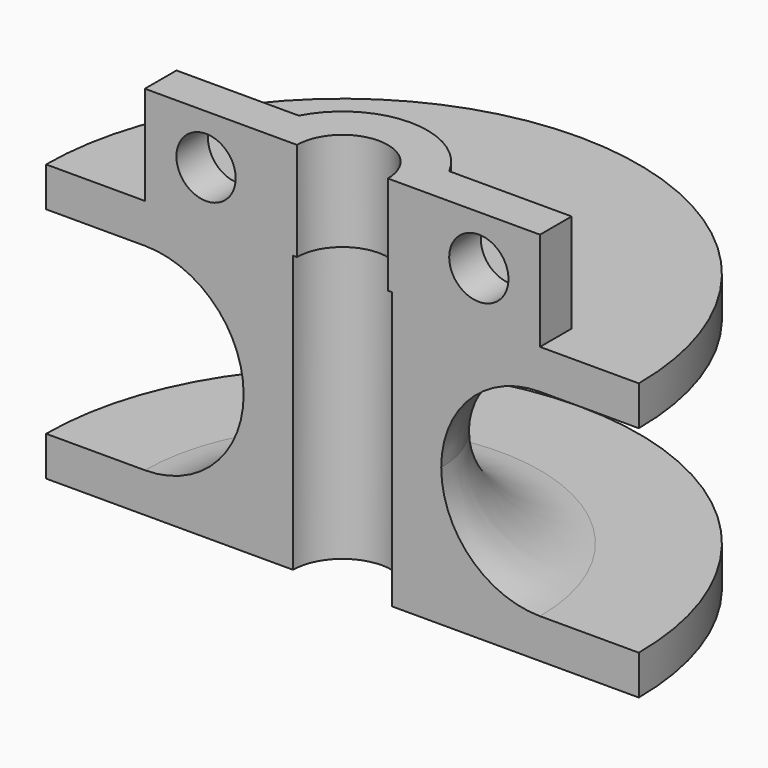
from build123d import *

# Parameters (mm, degrees)
F1_ANGLE = 180
F3_DEPTH = 5
F4_R     = 1.5
F5_DEPTH = 2.001
F6_R     = 4.99999


# Not quite as in the source:
# - a fillet or chamfer is up to 0.001 mm smaller than in the source, because OpenCascade refuses the exact size


with BuildPart() as f1:
    # F0 (on Front) → F1 (revolve)
    with BuildSketch(Plane.XZ):
        Polygon((-2.5, -7), (-2.5, 7), (-15, 7), (-15, 5), (-5, 5), (-5, -5), (-15, -5), (-15, -7), align=None)
    revolve(axis=Axis((0, 0, 0.6770828075), (0, 0, -1)), revolution_arc=F1_ANGLE)

    # F2 (on face) → F3 (join)
    with BuildSketch(Plane.XY.offset(7)):
        with BuildLine():
            Line((-10, 2), (-10, 0))
            Line((-10, 0), (-2.3, 0))
            ThreePointArc((-2.3, 0), (0, 2.3), (2.3, 0))
            Line((2.3, 0), (10, 0))
            Line((10, 0), (10, 2))
            Line((10, 2), (3.8065732621, 2))
            ThreePointArc((3.8065732621, 2), (0, 4.3), (-3.8065732621, 2))
            Line((-3.8065732621, 2), (-10, 2))
        make_face()
    extrude(amount=F3_DEPTH)

    # F4 (on face) → F5 (cut, through all)
    with BuildSketch(Plane(origin=(0, 2, 0), x_dir=(-1, 0, 0), z_dir=(0, 1, 0))):
        with Locations((6.9032866311, 9.5)):
            Circle(F4_R)
        with Locations((-6.9032866311, 9.5)):
            Circle(F4_R)
    extrude(amount=-F5_DEPTH, mode=Mode.SUBTRACT)

    # F6 (radius 5 in the source; OpenCascade refuses exactly that, so slightly less here)
    f6_edges = [f1.edges().sort_by_distance(p)[0] for p in [
        (0, 5, 5),
        (0, 5, -5),
    ]]
    fillet(f6_edges, radius=F6_R)


solid = f1.part
